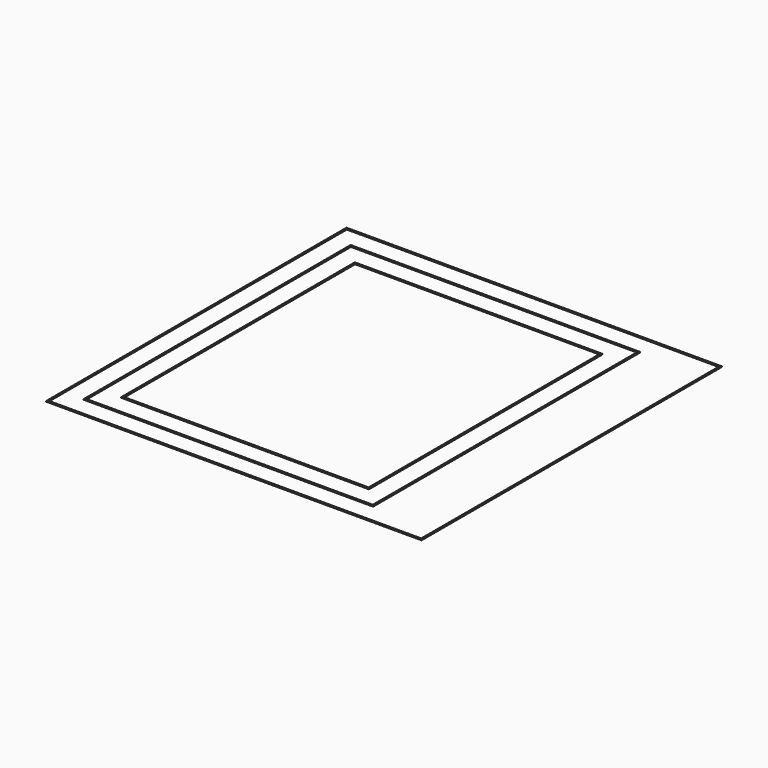
from build123d import *

# Parameters (mm, degrees)
F1_W     = 117
F1_H     = 117
F1_W_2   = 116
F1_H_2   = 116
F2_DEPTH = 0.2
F1_W_3   = 90.2133469
F1_H_3   = 104
F1_W_4   = 89.2133469
F1_H_4   = 103
F1_W_5   = 77.2133469
F1_H_5   = 91
F1_W_6   = 76.2133469
F1_H_6   = 90


# Not quite as in the source:
# - a feature names something its author has since deleted; it is built from what else it names


with BuildPart() as f2:
    # F1 (on Top) → F2 (new body)
    with BuildSketch(Plane.XY):
        with Locations((-32.9824382961, -13.6367691362)):
            Rectangle(F1_W, F1_H)
        with Locations((-32.9824382961, -13.6367691362)):
            Rectangle(F1_W_2, F1_H_2, mode=Mode.SUBTRACT)
    extrude(amount=F2_DEPTH)


with BuildPart() as f2b:
    # F1 (on Top) → F2, piece 2 (new body)
    with BuildSketch(Plane.XY):
        with Locations((-39.8757648461, -13.6367691362)):
            Rectangle(F1_W_3, F1_H_3)
        with Locations((-39.8757648461, -13.6367691362)):
            Rectangle(F1_W_4, F1_H_4, mode=Mode.SUBTRACT)
    extrude(amount=F2_DEPTH)


with BuildPart() as f2c:
    # F1 (on Top) → F2, piece 3 (new body)
    with BuildSketch(Plane.XY):
        with Locations((-39.8757648461, -13.6367691362)):
            Rectangle(F1_W_5, F1_H_5)
        with Locations((-39.8757648461, -13.6367691362)):
            Rectangle(F1_W_6, F1_H_6, mode=Mode.SUBTRACT)
    extrude(amount=F2_DEPTH)


solid = Compound([f2.part, f2b.part, f2c.part])
